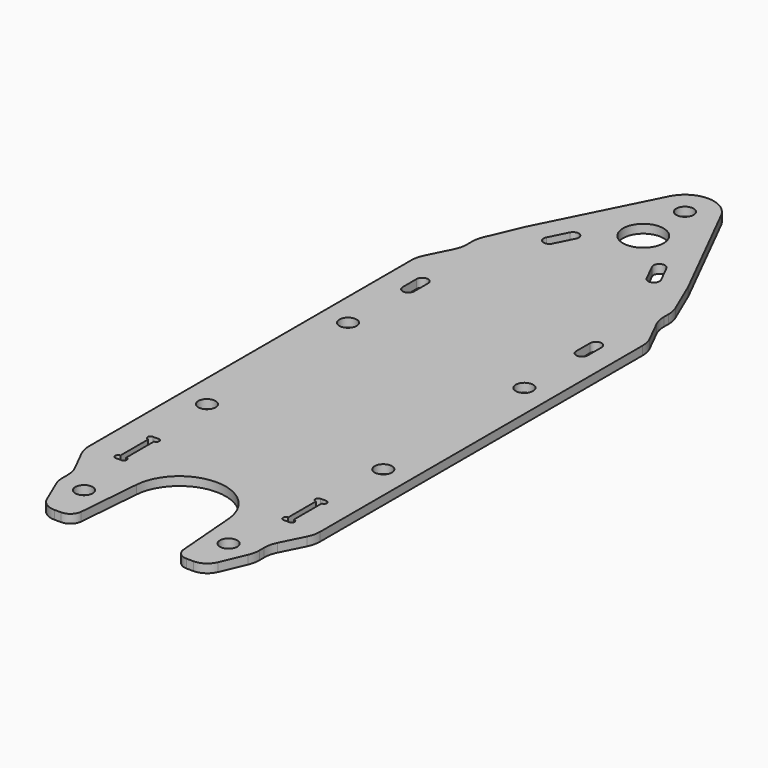
from build123d import *

# Parameters (mm, degrees)
F0_R        = 1.5
F0_R_2      = 3.5
F1_DEPTH    = 1.5
F2_T1_DEPTH = 1.5
F2_T3_DEPTH = 6.6314425489
F2_T5_DEPTH = 7.4016994375
F2_T7_DEPTH = 2.253003807
F4_DEPTH    = 25
F5_R        = 2
F6_R        = 3


# Not quite as in the source:
# - a fillet or chamfer that OpenCascade refuses, or shapes differently, is made with other operations: its cross-section is extruded or revolved along the edge and cut away or added


with BuildPart() as f1:
    # F0 (on Top) → F1 (new body)
    with BuildSketch(Plane.XY):
        with BuildLine():
            Line((-17, 42), (-20, 36))
            Line((-20, 36), (-20, -36))
            Line((-20, -36), (-17, -42))
            Line((-17, -42), (-17, -45.25))
            Line((-17, -45.25), (-14, -52.25))
            Line((-14, -52.25), (-9, -52.25))
            Line((-9, -52.25), (-7.9737930839, -39.6029885204))
            ThreePointArc((-7.9737930839, -39.6029885204), (0, -32.25), (7.9737930839, -39.6029885204))
            Line((7.9737930839, -39.6029885204), (9, -52.25))
            Line((9, -52.25), (14, -52.25))
            Line((14, -52.25), (17, -45.25))
            Line((17, -45.25), (17, -42))
            Line((17, -42), (20, -36))
            Line((20, -36), (20, 36))
            Line((20, 36), (17, 42))
            Line((17, 42), (17, 45.25))
            Line((17, 45.25), (14, 52.25))
            Line((14, 52.25), (4.468852459, 71.2426229508))
            ThreePointArc((4.468852459, 71.2426229508), (0, 74), (-4.468852459, 71.2426229508))
            Line((-4.468852459, 71.2426229508), (-14, 52.25))
            Line((-14, 52.25), (-17, 45.25))
            Line((-17, 45.25), (-17, 42))
        make_face()
        with Locations((-12.5, -45.25)):
            Circle(F0_R, mode=Mode.SUBTRACT)
        with Locations((-15.25, -15.25)):
            Circle(F0_R, mode=Mode.SUBTRACT)
        with Locations((12.5, -45.25)):
            Circle(F0_R, mode=Mode.SUBTRACT)
        with Locations((15.25, -15.25)):
            Circle(F0_R, mode=Mode.SUBTRACT)
        with Locations((-15.25, 15.25)):
            Circle(F0_R, mode=Mode.SUBTRACT)
        with BuildLine():
            Line((-16, 28), (-16, 31))
            ThreePointArc((-16, 31), (-15, 32), (-14, 31))
            Line((-14, 31), (-14, 28))
            ThreePointArc((-14, 28), (-15, 27), (-16, 28))
        make_face(mode=Mode.SUBTRACT)
        with BuildLine():
            Line((-6.5694088498, 53.6796721311), (-8.1392449154, 50.5514754098))
            ThreePointArc((-8.1392449154, 50.5514754098), (-9.4815399974, 50.1062295082), (-9.926785899, 51.4485245902))
            Line((-9.926785899, 51.4485245902), (-8.3569498334, 54.5767213115))
            ThreePointArc((-8.3569498334, 54.5767213115), (-7.0146547515, 55.0219672131), (-6.5694088498, 53.6796721311))
        make_face(mode=Mode.SUBTRACT)
        with Locations((15.25, 15.25)):
            Circle(F0_R, mode=Mode.SUBTRACT)
        with BuildLine():
            ThreePointArc((16, 28), (15, 27), (14, 28))
            Line((14, 28), (14, 31))
            ThreePointArc((14, 31), (15, 32), (16, 31))
            Line((16, 31), (16, 28))
        make_face(mode=Mode.SUBTRACT)
        with BuildLine():
            ThreePointArc((9.926785899, 51.4485245902), (9.4815399974, 50.1062295082), (8.1392449154, 50.5514754098))
            Line((8.1392449154, 50.5514754098), (6.5694088498, 53.6796721311))
            ThreePointArc((6.5694088498, 53.6796721311), (7.0146547515, 55.0219672131), (8.3569498334, 54.5767213115))
            Line((8.3569498334, 54.5767213115), (9.926785899, 51.4485245902))
        make_face(mode=Mode.SUBTRACT)
        with Locations((0, 60)):
            Circle(F0_R_2, mode=Mode.SUBTRACT)
        with Locations((0, 69)):
            Circle(F0_R, mode=Mode.SUBTRACT)
    extrude(amount=F1_DEPTH)

    # F2: fillet of radius 5 on 14 edges, made by hand

    # F2_s2 → F2_t1 (join)
    with BuildSketch(Plane.XY):
        with BuildLine():
            ThreePointArc((-17, 43.1803398875), (-17.1337550527, 42.0315752848), (-17.527864045, 40.94427191))
            Line((-17.527864045, 40.94427191), (-17, 42))
            Line((-17, 42), (-17, 43.1803398875))
        make_face()
        with BuildLine():
            ThreePointArc((17.527864045, 40.94427191), (17.1337550527, 42.0315752848), (17, 43.1803398875))
            Line((17, 43.1803398875), (17, 42))
            Line((17, 42), (17.527864045, 40.94427191))
        make_face()
        with BuildLine():
            ThreePointArc((17, -43.1803398875), (17.1337550527, -42.0315752848), (17.527864045, -40.94427191))
            Line((17.527864045, -40.94427191), (17, -42))
            Line((17, -42), (17, -43.1803398875))
        make_face()
        with BuildLine():
            ThreePointArc((-17.527864045, -40.94427191), (-17.1337550527, -42.0315752848), (-17, -43.1803398875))
            Line((-17, -43.1803398875), (-17, -42))
            Line((-17, -42), (-17.527864045, -40.94427191))
        make_face()
    extrude(amount=F2_T1_DEPTH)

    # F2_s4 → F2_t3 (cut)
    with BuildSketch(Plane.XY.offset(-2.5657212744)):
        with BuildLine():
            ThreePointArc((16.5957251501, -46.1933079831), (16.897888614, -45.2290408516), (17, -44.2237114902))
            Line((17, -44.2237114902), (17, -45.25))
            Line((17, -45.25), (16.5957251501, -46.1933079831))
        make_face()
        with BuildLine():
            ThreePointArc((-16.5957251501, 46.1933079831), (-16.897888614, 45.2290408516), (-17, 44.2237114902))
            Line((-17, 44.2237114902), (-17, 45.25))
            Line((-17, 45.25), (-16.5957251501, 46.1933079831))
        make_face()
        with BuildLine():
            ThreePointArc((16.5957251501, 46.1933079831), (16.897888614, 45.2290408516), (17, 44.2237114902))
            Line((17, 44.2237114902), (17, 45.25))
            Line((17, 45.25), (16.5957251501, 46.1933079831))
        make_face()
        with BuildLine():
            ThreePointArc((-17, -44.2237114902), (-16.897888614, -45.2290408516), (-16.5957251501, -46.1933079831))
            Line((-16.5957251501, -46.1933079831), (-17, -45.25))
            Line((-17, -45.25), (-17, -44.2237114902))
        make_face()
    extrude(amount=F2_T3_DEPTH, mode=Mode.SUBTRACT)

    # F2_s6 → F2_t5 (cut)
    with BuildSketch(Plane.XY.offset(-2.9508497187)):
        with BuildLine():
            ThreePointArc((-19.472135955, 37.05572809), (-19.8662449473, 35.9684247152), (-20, 34.8196601125))
            Line((-20, 34.8196601125), (-20, 36))
            Line((-20, 36), (-19.472135955, 37.05572809))
        make_face()
        with BuildLine():
            ThreePointArc((20, 34.8196601125), (19.8662449473, 35.9684247152), (19.472135955, 37.05572809))
            Line((19.472135955, 37.05572809), (20, 36))
            Line((20, 36), (20, 34.8196601125))
        make_face()
        with BuildLine():
            ThreePointArc((19.472135955, -37.05572809), (19.8662449473, -35.9684247152), (20, -34.8196601125))
            Line((20, -34.8196601125), (20, -36))
            Line((20, -36), (19.472135955, -37.05572809))
        make_face()
        with BuildLine():
            ThreePointArc((-20, -34.8196601125), (-19.8662449473, -35.9684247152), (-19.472135955, -37.05572809))
            Line((-19.472135955, -37.05572809), (-20, -36))
            Line((-20, -36), (-20, -34.8196601125))
        make_face()
    extrude(amount=F2_T5_DEPTH, mode=Mode.SUBTRACT)

    # F2_s8 → F2_t7 (cut)
    with BuildSketch(Plane.XY.offset(-0.3765019035)):
        with BuildLine():
            ThreePointArc((-13.9324518552, 52.3846025166), (-13.9979436343, 52.2490444272), (-14.0593245463, 52.1115760587))
            Line((-14.0593245463, 52.1115760587), (-14, 52.25))
            Line((-14, 52.25), (-13.9324518552, 52.3846025166))
        make_face()
        with BuildLine():
            ThreePointArc((13.9324518552, 52.3846025166), (13.9979436343, 52.2490444272), (14.0593245463, 52.1115760587))
            Line((14.0593245463, 52.1115760587), (14, 52.25))
            Line((14, 52.25), (13.9324518552, 52.3846025166))
        make_face()
    extrude(amount=F2_T7_DEPTH, mode=Mode.SUBTRACT)

    # F3 (on face) → F4 (cut)
    with BuildSketch(Plane.XY.offset(1.5)):
        with BuildLine():
            Line((-14, -27.25), (-15, -27.25))
            ThreePointArc((-15, -27.25), (-15.5, -27.75), (-15, -28.25))
            Line((-15, -28.25), (-15, -34.25))
            ThreePointArc((-15, -34.25), (-15.5, -34.75), (-15, -35.25))
            Line((-15, -35.25), (-14, -35.25))
            ThreePointArc((-14, -35.25), (-13.5, -34.75), (-14, -34.25))
            Line((-14, -34.25), (-14, -28.25))
            ThreePointArc((-14, -28.25), (-13.5, -27.75), (-14, -27.25))
        make_face()
        with BuildLine():
            Line((14, -35.25), (15, -35.25))
            ThreePointArc((15, -35.25), (15.5, -34.75), (15, -34.25))
            Line((15, -34.25), (15, -28.25))
            ThreePointArc((15, -28.25), (15.5, -27.75), (15, -27.25))
            Line((15, -27.25), (14, -27.25))
            ThreePointArc((14, -27.25), (13.5, -27.75), (14, -28.25))
            Line((14, -28.25), (14, -34.25))
            ThreePointArc((14, -34.25), (13.5, -34.75), (14, -35.25))
        make_face()
    extrude(amount=-F4_DEPTH, mode=Mode.SUBTRACT)

    # F5
    f5_edges = [f1.edges().sort_by_distance(p)[0] for p in [
        (-9, -52.25, 0.75),
        (9, -52.25, 0.75),
    ]]
    fillet(f5_edges, radius=F5_R)

    # F6
    f6_edges = [f1.edges().sort_by_distance(p)[0] for p in [
        (-14, -52.25, 0.75),
        (14, -52.25, 0.75),
    ]]
    fillet(f6_edges, radius=F6_R)


solid = f1.part
